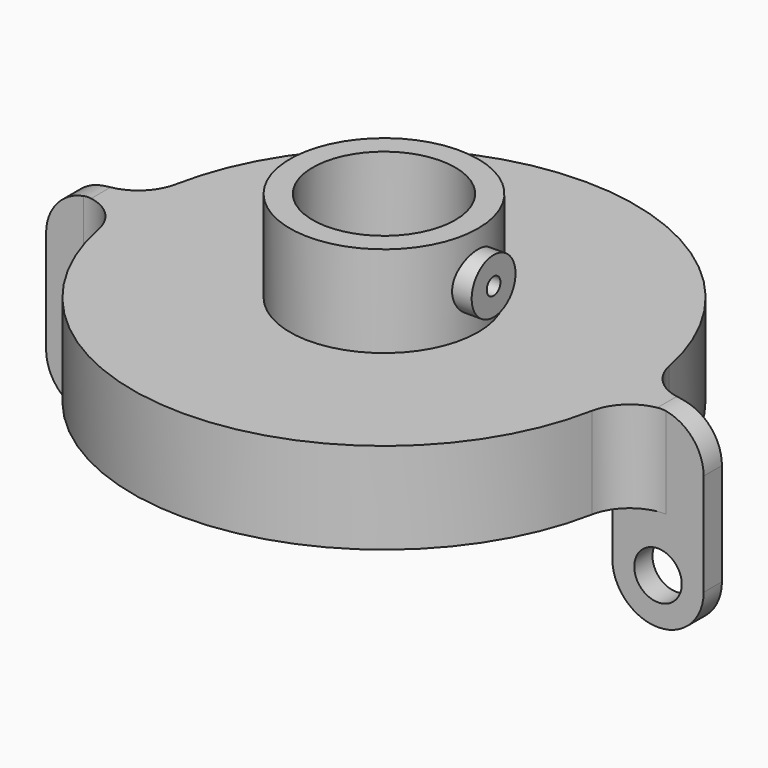
from build123d import *

# Parameters (mm, degrees)
F0_R      = 17.4625
F1_DEPTH  = 6.35
F2_R      = 16.51
F3_DEPTH  = 4.7625
F4_R      = 3.81
F5_DEPTH  = 6.351
F6_W      = 6.35
F6_H      = 13.462
F7_DEPTH  = 0.79375
F9_R      = 3.17499
F10_R     = 3.175
F11_R     = 1.651
F12_DEPTH = 18.25725
F13_R     = 6.5405
F13_R_2   = 4.953
F14_DEPTH = 6.35
F16_R     = 1.905
F17_DEPTH = 1.3630747169
F18_R     = 0.59563
F19_DEPTH = 2.7039446902


# Not quite as in the source:
# - a fillet or chamfer is up to 0.001 mm smaller than in the source, because OpenCascade refuses the exact size


with BuildPart() as f1:
    # F0 (on Top) → F1 (new body)
    with BuildSketch(Plane.XY):
        Circle(F0_R)
    extrude(amount=F1_DEPTH)

    # F2 (on face) → F3 (cut)
    with BuildSketch(Plane(origin=(0, 0, 0), x_dir=(1, 0, 0), z_dir=(0, 0, -1))):
        Circle(F2_R)
    extrude(amount=-F3_DEPTH, mode=Mode.SUBTRACT)

    # F4 (on face) → F5 (cut, through all)
    with BuildSketch(Plane.XY.offset(6.35)):
        Circle(F4_R)
    extrude(amount=-F5_DEPTH, mode=Mode.SUBTRACT)

    # F6 (on Front) → F7 (join, symmetric)
    with BuildSketch(Plane.XZ):
        with Locations((-19.685, -0.381)):
            Rectangle(F6_W, F6_H)
    extrude(amount=F7_DEPTH, both=True)

    # F8: F1 across plane


with BuildPart() as f1_1:
    add(f1.part)
    add(f1.part.mirror(Plane.YZ))

    # F9 (radius 3.175 in the source; OpenCascade refuses exactly that, so slightly less here)
    f9_edges = [f1_1.edges().sort_by_distance(p)[0] for p in [
        (-22.86, 0, 6.35),
        (-22.86, 0, -7.112),
        (-16.51, 0, -7.112),
        (22.86, 0, 6.35),
        (22.86, 0, -7.112),
        (16.51, 0, -7.112),
    ]]
    fillet(f9_edges, radius=F9_R)

    # F10 (call 1 of 4: OpenCascade refuses the feature's edges together)
    f10_edges = [f1_1.edges().sort_by_distance(p)[0] for p in [
        (-17.444451, -0.79375, 3.175),
    ]]
    fillet(f10_edges, radius=F10_R)

    # F10#2 (call 2 of 4)
    f10_2_edges = [f1_1.edges().sort_by_distance(p)[0] for p in [
        (-17.444451, 0.79375, 3.175),
    ]]
    fillet(f10_2_edges, radius=F10_R)

    # F10#3 (call 3 of 4)
    f10_3_edges = [f1_1.edges().sort_by_distance(p)[0] for p in [
        (17.444451, -0.79375, 3.175),
    ]]
    fillet(f10_3_edges, radius=F10_R)

    # F10#4 (call 4 of 4)
    f10_4_edges = [f1_1.edges().sort_by_distance(p)[0] for p in [
        (17.444451, 0.79375, 3.175),
    ]]
    fillet(f10_4_edges, radius=F10_R)

    # F11 (on face) → F12 (cut, through all)
    with BuildSketch(Plane(origin=(0, 0.79375, 0), x_dir=(-1, 0, 0), z_dir=(0, 1, 0))):
        with Locations((19.685, -3.937)):
            Circle(F11_R)
        with Locations((-19.685, -3.937)):
            Circle(F11_R)
    extrude(amount=-F12_DEPTH, mode=Mode.SUBTRACT)

    # F13 (on face) → F14 (join)
    with BuildSketch(Plane.XY.offset(6.35)):
        Circle(F13_R)
        Circle(F13_R_2, mode=Mode.SUBTRACT)
    extrude(amount=F14_DEPTH)

    # F16 (on offset) → F17 (join, through all)
    with BuildSketch(Plane.YZ.offset(7.62)):
        with Locations((0, 9.525)):
            Circle(F16_R)
    extrude(amount=-F17_DEPTH)

    # F18 (on face) → F19 (cut, through all)
    with BuildSketch(Plane.YZ.offset(7.62)):
        with Locations((0, 9.525)):
            Circle(F18_R)
    extrude(amount=-F19_DEPTH, mode=Mode.SUBTRACT)


solid = f1_1.part
